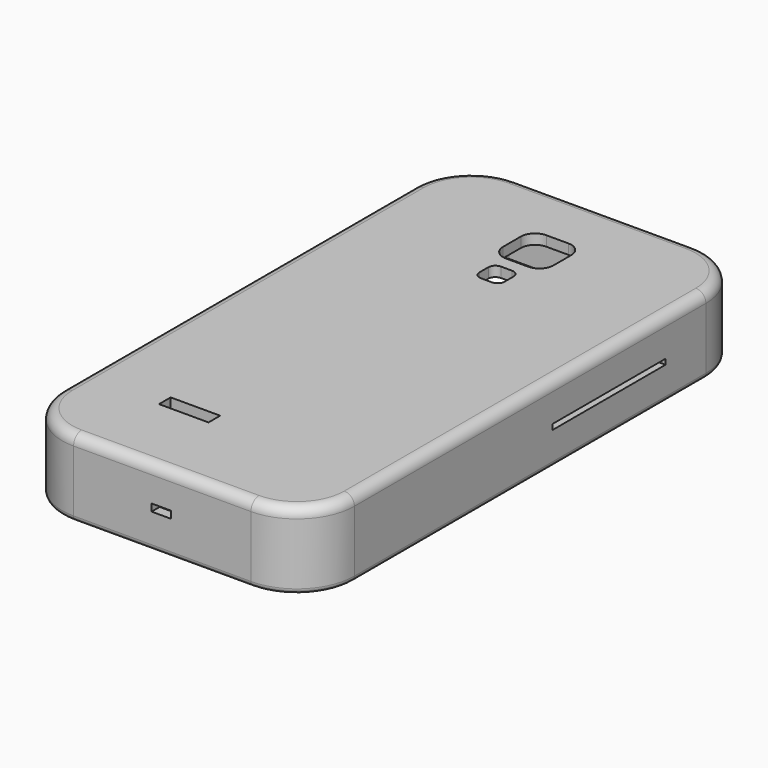
from build123d import *

# Parameters (mm, degrees)
F1_DEPTH   = 14.224
F2_W       = 16.002
F2_H       = 1.3465428281
F2_W_2     = 9.398
F2_W_3     = 10.16
F3_DEPTH   = 76.2
F4_W       = 13.4153888345
F4_H       = 1.2321065667
F5_DEPTH   = 25.4
F7_DEPTH   = 14.224
F1_FACE2_W = 12.4812044669
F1_FACE2_H = 3.6749392748
F8_DEPTH   = 2.54
F9_DEPTH   = 2.54
F11_R      = 1.27
F6_W       = 4.8780030338
F6_H       = 1.8081708086
F12_DEPTH  = 7.1882
F13_R      = 2.54


with BuildPart() as f1:
    # F0 (on Top) → F1 (new body)
    with BuildSketch(Plane.XY):
        with BuildLine():
            Line((1.0885104024, 77.2395779495), (-21.2634895976, 77.2395779495))
            ThreePointArc((-21.2634895976, 77.2395779495), (-29.7049303514, 73.7430187033), (-33.2014895976, 65.3015779495))
            Line((-33.2014895976, 65.3015779495), (-33.2014895976, -45.4424220505))
            ThreePointArc((-33.2014895976, -45.4424220505), (-29.7049303514, -53.8838628043), (-21.2634895976, -57.3804220505))
            Line((-21.2634895976, -57.3804220505), (1.0885104024, -57.3804220505))
            Line((1.0885104024, -57.3804220505), (1.0885104024, -54.8404220505))
            Line((1.0885104024, -54.8404220505), (-21.2634895976, -54.8404220505))
            ThreePointArc((-21.2634895976, -54.8404220505), (-27.9088791272, -52.0878115801), (-30.6614895976, -45.4424220505))
            Line((-30.6614895976, -45.4424220505), (-30.6614895976, 65.3015779495))
            ThreePointArc((-30.6614895976, 65.3015779495), (-27.9088791272, 71.9469674791), (-21.2634895976, 74.6995779495))
            Line((-21.2634895976, 74.6995779495), (1.0885104024, 74.6995779495))
            Line((1.0885104024, 74.6995779495), (1.0885104024, 77.2395779495))
        make_face()
        with BuildLine():
            Line((23.4405104024, 77.2395779495), (1.0885104024, 77.2395779495))
            Line((1.0885104024, 77.2395779495), (1.0885104024, 74.6995779495))
            Line((1.0885104024, 74.6995779495), (23.4405104024, 74.6995779495))
            ThreePointArc((23.4405104024, 74.6995779495), (30.085899932, 71.9469674791), (32.8385104024, 65.3015779495))
            Line((32.8385104024, 65.3015779495), (32.8385104024, -45.4424220505))
            ThreePointArc((32.8385104024, -45.4424220505), (30.085899932, -52.0878115801), (23.4405104024, -54.8404220505))
            Line((23.4405104024, -54.8404220505), (1.0885104024, -54.8404220505))
            Line((1.0885104024, -54.8404220505), (1.0885104024, -57.3804220505))
            Line((1.0885104024, -57.3804220505), (23.4405104024, -57.3804220505))
            ThreePointArc((23.4405104024, -57.3804220505), (31.8819511562, -53.8838628043), (35.3785104024, -45.4424220505))
            Line((35.3785104024, -45.4424220505), (35.3785104024, 65.3015779495))
            ThreePointArc((35.3785104024, 65.3015779495), (31.8819511562, 73.7430187033), (23.4405104024, 77.2395779495))
        make_face()
        with BuildLine():
            Line((23.4405104024, 74.6995779495), (1.0885104024, 74.6995779495))
            Line((1.0885104024, 74.6995779495), (1.0885104024, 64.5395779495))
            Line((1.0885104024, 64.5395779495), (3.8825104024, 64.5395779495))
            ThreePointArc((3.8825104024, 64.5395779495), (6.3969821163, 63.4980496634), (7.4385104024, 60.9835779495))
            Line((7.4385104024, 60.9835779495), (7.4385104024, 55.3955779495))
            ThreePointArc((7.4385104024, 55.3955779495), (6.3969821163, 52.8811062356), (3.8825104024, 51.8395779495))
            Line((3.8825104024, 51.8395779495), (1.0885104024, 51.8395779495))
            Line((1.0885104024, 51.8395779495), (1.0885104024, 48.5375779495))
            Line((1.0885104024, 48.5375779495), (2.4855104024, 48.5375779495))
            ThreePointArc((2.4855104024, 48.5375779495), (3.7427462594, 48.0168138065), (4.2635104024, 46.7595779495))
            Line((4.2635104024, 46.7595779495), (4.2635104024, 43.9655779495))
            ThreePointArc((4.2635104024, 43.9655779495), (3.7427462594, 42.7083420926), (2.4855104024, 42.1875779495))
            Line((2.4855104024, 42.1875779495), (1.0885104024, 42.1875779495))
            Line((1.0885104024, 42.1875779495), (1.0885104024, -54.8404220505))
            Line((1.0885104024, -54.8404220505), (23.4405104024, -54.8404220505))
            ThreePointArc((23.4405104024, -54.8404220505), (30.085899932, -52.0878115801), (32.8385104024, -45.4424220505))
            Line((32.8385104024, -45.4424220505), (32.8385104024, 65.3015779495))
            ThreePointArc((32.8385104024, 65.3015779495), (30.085899932, 71.9469674791), (23.4405104024, 74.6995779495))
        make_face()
        with BuildLine():
            Line((1.0885104024, 64.5395779495), (1.0885104024, 74.6995779495))
            Line((1.0885104024, 74.6995779495), (-21.2634895976, 74.6995779495))
            ThreePointArc((-21.2634895976, 74.6995779495), (-27.9088791272, 71.9469674791), (-30.6614895976, 65.3015779495))
            Line((-30.6614895976, 65.3015779495), (-30.6614895976, -45.4424220505))
            ThreePointArc((-30.6614895976, -45.4424220505), (-27.9088791272, -52.0878115801), (-21.2634895976, -54.8404220505))
            Line((-21.2634895976, -54.8404220505), (1.0885104024, -54.8404220505))
            Line((1.0885104024, -54.8404220505), (1.0885104024, 42.1875779495))
            Line((1.0885104024, 42.1875779495), (-0.3084895976, 42.1875779495))
            ThreePointArc((-0.3084895976, 42.1875779495), (-1.5657254545, 42.7083420926), (-2.0864895976, 43.9655779495))
            Line((-2.0864895976, 43.9655779495), (-2.0864895976, 46.7595779495))
            ThreePointArc((-2.0864895976, 46.7595779495), (-1.5657254545, 48.0168138065), (-0.3084895976, 48.5375779495))
            Line((-0.3084895976, 48.5375779495), (1.0885104024, 48.5375779495))
            Line((1.0885104024, 48.5375779495), (1.0885104024, 51.8395779495))
            Line((1.0885104024, 51.8395779495), (-1.7054895976, 51.8395779495))
            ThreePointArc((-1.7054895976, 51.8395779495), (-4.2199613115, 52.8811062356), (-5.2614895976, 55.3955779495))
            Line((-5.2614895976, 55.3955779495), (-5.2614895976, 60.9835779495))
            ThreePointArc((-5.2614895976, 60.9835779495), (-4.2199613115, 63.4980496634), (-1.7054895976, 64.5395779495))
            Line((-1.7054895976, 64.5395779495), (1.0885104024, 64.5395779495))
        make_face()
        Polygon((-16.2484161556, -39.2828993499), (-16.2484161556, -37.4030255506), (-16.2484161556, -35.6079600751), (-3.7672116887, -35.6079600751), (-3.7672116887, -39.2828993499), align=None, mode=Mode.SUBTRACT)
    extrude(amount=F1_DEPTH)

    # F2 (on face) → F3 (join)
    with BuildSketch(Plane(origin=(-33.2014895976, 0, 0), x_dir=(0, -1, 0), z_dir=(-1, 0, 0))):
        with Locations((-44.6005779495, 6.438728586)):
            Rectangle(F2_W, F2_H)
        with Locations((-31.9005779495, 6.438728586)):
            Rectangle(F2_W_2, F2_H)
        with Locations((-22.1215779495, 6.438728586)):
            Rectangle(F2_W_3, F2_H)
    extrude(amount=-F3_DEPTH)

    # F4 (on face) → F5 (join)
    with BuildSketch(Plane(origin=(-33.2014895976, 0, 0), x_dir=(0, -1, 0), z_dir=(-1, 0, 0))):
        with Locations((-33.9092723668, 6.4959467167)):
            Rectangle(F4_W, F4_H)
    extrude(amount=F5_DEPTH)


with BuildPart() as f7:
    # F0 (on Top) → F7 (new body)
    with BuildSketch(Plane.XY):
        with BuildLine():
            Line((37.9185104024, -45.4424220505), (37.9185104024, 65.3015779495))
            ThreePointArc((37.9185104024, 65.3015779495), (33.6780023805, 75.5390699275), (23.4405104024, 79.7795779495))
            Line((23.4405104024, 79.7795779495), (-21.2634895976, 79.7795779495))
            ThreePointArc((-21.2634895976, 79.7795779495), (-31.5009815756, 75.5390699275), (-35.7414895976, 65.3015779495))
            Line((-35.7414895976, 65.3015779495), (-35.7414895976, -45.4424220505))
            ThreePointArc((-35.7414895976, -45.4424220505), (-31.5009815756, -55.6799140285), (-21.2634895976, -59.9204220505))
            Line((-21.2634895976, -59.9204220505), (23.4405104024, -59.9204220505))
            ThreePointArc((23.4405104024, -59.9204220505), (33.6780023805, -55.6799140285), (37.9185104024, -45.4424220505))
        make_face()
        with BuildLine():
            ThreePointArc((-33.2014895976, 65.3015779495), (-29.7049303514, 73.7430187033), (-21.2634895976, 77.2395779495))
            Line((-21.2634895976, 77.2395779495), (1.0885104024, 77.2395779495))
            Line((1.0885104024, 77.2395779495), (23.4405104024, 77.2395779495))
            ThreePointArc((23.4405104024, 77.2395779495), (31.8819511562, 73.7430187033), (35.3785104024, 65.3015779495))
            Line((35.3785104024, 65.3015779495), (35.3785104024, -45.4424220505))
            ThreePointArc((35.3785104024, -45.4424220505), (31.8819511562, -53.8838628043), (23.4405104024, -57.3804220505))
            Line((23.4405104024, -57.3804220505), (1.0885104024, -57.3804220505))
            Line((1.0885104024, -57.3804220505), (-21.2634895976, -57.3804220505))
            ThreePointArc((-21.2634895976, -57.3804220505), (-29.7049303514, -53.8838628043), (-33.2014895976, -45.4424220505))
            Line((-33.2014895976, -45.4424220505), (-33.2014895976, 65.3015779495))
        make_face(mode=Mode.SUBTRACT)
    extrude(amount=F7_DEPTH)

    # F7_face (on face) + F1_face2 (on face) → F8 (join)
    with BuildSketch(Plane(origin=(1.0885104024, 9.9295779495, 14.224), x_dir=(1, 0, 0), z_dir=(0, 0, 1))):
        with BuildLine():
            ThreePointArc((22.352, -69.85), (32.589491978, -65.609491978), (36.83, -55.372))
            Line((36.83, -55.372), (36.83, 55.372))
            ThreePointArc((36.83, 55.372), (32.589491978, 65.609491978), (22.352, 69.85))
            Line((22.352, 69.85), (-22.352, 69.85))
            ThreePointArc((-22.352, 69.85), (-32.589491978, 65.609491978), (-36.83, 55.372))
            Line((-36.83, 55.372), (-36.83, -55.372))
            ThreePointArc((-36.83, -55.372), (-32.589491978, -65.609491978), (-22.352, -69.85))
            Line((-22.352, -69.85), (22.352, -69.85))
        make_face()
        with BuildLine():
            ThreePointArc((-34.29, 55.372), (-30.7934407538, 63.8134407538), (-22.352, 67.31))
            Line((-22.352, 67.31), (22.352, 67.31))
            ThreePointArc((22.352, 67.31), (30.7934407538, 63.8134407538), (34.29, 55.372))
            Line((34.29, 55.372), (34.29, -55.372))
            ThreePointArc((34.29, -55.372), (30.7934407538, -63.8134407538), (22.352, -67.31))
            Line((22.352, -67.31), (-22.352, -67.31))
            ThreePointArc((-22.352, -67.31), (-30.7934407538, -63.8134407538), (-34.29, -55.372))
            Line((-34.29, -55.372), (-34.29, 55.372))
        make_face(mode=Mode.SUBTRACT)
    with BuildSketch(Plane(origin=(1.1458518889, 9.2063211199, 14.224), x_dir=(1, 0, 0), z_dir=(0, 0, 1))):
        with BuildLine():
            ThreePointArc((-22.4093414865, 68.0332568296), (-30.8507822403, 64.5366975834), (-34.3473414865, 56.0952568296))
            Line((-34.3473414865, 56.0952568296), (-34.3473414865, -54.6487431704))
            ThreePointArc((-34.3473414865, -54.6487431704), (-30.8507822403, -63.0901839242), (-22.4093414865, -66.5867431704))
            Line((-22.4093414865, -66.5867431704), (22.2946585135, -66.5867431704))
            ThreePointArc((22.2946585135, -66.5867431704), (30.7360992673, -63.0901839242), (34.2326585135, -54.6487431704))
            Line((34.2326585135, -54.6487431704), (34.2326585135, 56.0952568296))
            ThreePointArc((34.2326585135, 56.0952568296), (30.7360992673, 64.5366975834), (22.2946585135, 68.0332568296))
            Line((22.2946585135, 68.0332568296), (-22.4093414865, 68.0332568296))
        make_face()
        with BuildLine():
            ThreePointArc((2.7366585135, 55.3332568296), (5.2511302274, 54.2917285435), (6.2926585135, 51.7772568296))
            Line((6.2926585135, 51.7772568296), (6.2926585135, 46.1892568296))
            ThreePointArc((6.2926585135, 46.1892568296), (5.2511302274, 43.6747851157), (2.7366585135, 42.6332568296))
            Line((2.7366585135, 42.6332568296), (-2.8513414865, 42.6332568296))
            ThreePointArc((-2.8513414865, 42.6332568296), (-5.3658132004, 43.6747851157), (-6.4073414865, 46.1892568296))
            Line((-6.4073414865, 46.1892568296), (-6.4073414865, 51.7772568296))
            ThreePointArc((-6.4073414865, 51.7772568296), (-5.3658132004, 54.2917285435), (-2.8513414865, 55.3332568296))
            Line((-2.8513414865, 55.3332568296), (2.7366585135, 55.3332568296))
        make_face(mode=Mode.SUBTRACT)
        with BuildLine():
            ThreePointArc((1.3396585135, 39.3312568296), (2.5968943705, 38.8104926866), (3.1176585135, 37.5532568296))
            Line((3.1176585135, 37.5532568296), (3.1176585135, 34.7592568296))
            ThreePointArc((3.1176585135, 34.7592568296), (2.5968943705, 33.5020209727), (1.3396585135, 32.9812568296))
            Line((1.3396585135, 32.9812568296), (-1.4543414865, 32.9812568296))
            ThreePointArc((-1.4543414865, 32.9812568296), (-2.7115773434, 33.5020209727), (-3.2323414865, 34.7592568296))
            Line((-3.2323414865, 34.7592568296), (-3.2323414865, 37.5532568296))
            ThreePointArc((-3.2323414865, 37.5532568296), (-2.7115773434, 38.8104926866), (-1.4543414865, 39.3312568296))
            Line((-1.4543414865, 39.3312568296), (1.3396585135, 39.3312568296))
        make_face(mode=Mode.SUBTRACT)
        with Locations((-11.1536658111, -46.6517508324)):
            Rectangle(F1_FACE2_W, F1_FACE2_H, mode=Mode.SUBTRACT)
    extrude(amount=F8_DEPTH)

    # F0 (on Top) → F9 (join)
    with BuildSketch(Plane.XY):
        with BuildLine():
            Line((37.9185104024, -45.4424220505), (37.9185104024, 65.3015779495))
            ThreePointArc((37.9185104024, 65.3015779495), (33.6780023805, 75.5390699275), (23.4405104024, 79.7795779495))
            Line((23.4405104024, 79.7795779495), (-21.2634895976, 79.7795779495))
            ThreePointArc((-21.2634895976, 79.7795779495), (-31.5009815756, 75.5390699275), (-35.7414895976, 65.3015779495))
            Line((-35.7414895976, 65.3015779495), (-35.7414895976, -45.4424220505))
            ThreePointArc((-35.7414895976, -45.4424220505), (-31.5009815756, -55.6799140285), (-21.2634895976, -59.9204220505))
            Line((-21.2634895976, -59.9204220505), (23.4405104024, -59.9204220505))
            ThreePointArc((23.4405104024, -59.9204220505), (33.6780023805, -55.6799140285), (37.9185104024, -45.4424220505))
        make_face()
        with BuildLine():
            ThreePointArc((-33.2014895976, 65.3015779495), (-29.7049303514, 73.7430187033), (-21.2634895976, 77.2395779495))
            Line((-21.2634895976, 77.2395779495), (1.0885104024, 77.2395779495))
            Line((1.0885104024, 77.2395779495), (23.4405104024, 77.2395779495))
            ThreePointArc((23.4405104024, 77.2395779495), (31.8819511562, 73.7430187033), (35.3785104024, 65.3015779495))
            Line((35.3785104024, 65.3015779495), (35.3785104024, -45.4424220505))
            ThreePointArc((35.3785104024, -45.4424220505), (31.8819511562, -53.8838628043), (23.4405104024, -57.3804220505))
            Line((23.4405104024, -57.3804220505), (1.0885104024, -57.3804220505))
            Line((1.0885104024, -57.3804220505), (-21.2634895976, -57.3804220505))
            ThreePointArc((-21.2634895976, -57.3804220505), (-29.7049303514, -53.8838628043), (-33.2014895976, -45.4424220505))
            Line((-33.2014895976, -45.4424220505), (-33.2014895976, 65.3015779495))
        make_face(mode=Mode.SUBTRACT)
        with BuildLine():
            Line((23.4405104024, 77.2395779495), (1.0885104024, 77.2395779495))
            Line((1.0885104024, 77.2395779495), (1.0885104024, 74.6995779495))
            Line((1.0885104024, 74.6995779495), (23.4405104024, 74.6995779495))
            ThreePointArc((23.4405104024, 74.6995779495), (30.085899932, 71.9469674791), (32.8385104024, 65.3015779495))
            Line((32.8385104024, 65.3015779495), (32.8385104024, -45.4424220505))
            ThreePointArc((32.8385104024, -45.4424220505), (30.085899932, -52.0878115801), (23.4405104024, -54.8404220505))
            Line((23.4405104024, -54.8404220505), (1.0885104024, -54.8404220505))
            Line((1.0885104024, -54.8404220505), (1.0885104024, -57.3804220505))
            Line((1.0885104024, -57.3804220505), (23.4405104024, -57.3804220505))
            ThreePointArc((23.4405104024, -57.3804220505), (31.8819511562, -53.8838628043), (35.3785104024, -45.4424220505))
            Line((35.3785104024, -45.4424220505), (35.3785104024, 65.3015779495))
            ThreePointArc((35.3785104024, 65.3015779495), (31.8819511562, 73.7430187033), (23.4405104024, 77.2395779495))
        make_face()
        with BuildLine():
            Line((1.0885104024, 77.2395779495), (-21.2634895976, 77.2395779495))
            ThreePointArc((-21.2634895976, 77.2395779495), (-29.7049303514, 73.7430187033), (-33.2014895976, 65.3015779495))
            Line((-33.2014895976, 65.3015779495), (-33.2014895976, -45.4424220505))
            ThreePointArc((-33.2014895976, -45.4424220505), (-29.7049303514, -53.8838628043), (-21.2634895976, -57.3804220505))
            Line((-21.2634895976, -57.3804220505), (1.0885104024, -57.3804220505))
            Line((1.0885104024, -57.3804220505), (1.0885104024, -54.8404220505))
            Line((1.0885104024, -54.8404220505), (-21.2634895976, -54.8404220505))
            ThreePointArc((-21.2634895976, -54.8404220505), (-27.9088791272, -52.0878115801), (-30.6614895976, -45.4424220505))
            Line((-30.6614895976, -45.4424220505), (-30.6614895976, 65.3015779495))
            ThreePointArc((-30.6614895976, 65.3015779495), (-27.9088791272, 71.9469674791), (-21.2634895976, 74.6995779495))
            Line((-21.2634895976, 74.6995779495), (1.0885104024, 74.6995779495))
            Line((1.0885104024, 74.6995779495), (1.0885104024, 77.2395779495))
        make_face()
    extrude(amount=-F9_DEPTH)

    # F10: cut F1
    add(f1.part, mode=Mode.SUBTRACT)

    # F11
    f11_edges = [f7.edges().sort_by_distance(p)[0] for p in [
        (-30.66149, 9.929578, -2.54),
        (-35.74149, 9.929578, -2.54),
        (33.678002, -55.679914, -2.54),
        (1.08851, -59.920422, -2.54),
        (37.91851, 9.929578, -2.54),
        (33.678002, 75.53907, -2.54),
        (1.08851, 79.779578, -2.54),
        (-31.500982, 75.53907, -2.54),
        (-31.500982, -55.679914, -2.54),
        (30.0859, 71.946967, -2.54),
        (32.83851, 9.929578, -2.54),
        (30.0859, -52.087812, -2.54),
        (1.08851, -54.840422, -2.54),
        (-27.908879, -52.087812, -2.54),
        (-27.908879, 71.946967, -2.54),
        (1.08851, 74.699578, -2.54),
    ]]
    fillet(f11_edges, radius=F11_R)

    # F6 (on face) → F12 (cut, symmetric)
    with BuildSketch(Plane.XZ.offset(57.3804220505)):
        with Locations((0.8325793897, 6.9699145957)):
            Rectangle(F6_W, F6_H)
    extrude(amount=F12_DEPTH, both=True, mode=Mode.SUBTRACT)

    # F13
    f13_edges = [f7.edges().sort_by_distance(p)[0] for p in [
        (37.91851, 9.929578, 16.764),
        (33.678002, -55.679914, 16.764),
        (1.08851, -59.920422, 16.764),
        (33.678002, 75.53907, 16.764),
        (1.08851, 79.779578, 16.764),
        (-31.500982, 75.53907, 16.764),
        (-35.74149, 9.929578, 16.764),
        (-31.500982, -55.679914, 16.764),
    ]]
    fillet(f13_edges, radius=F13_R)


solid = f7.part
